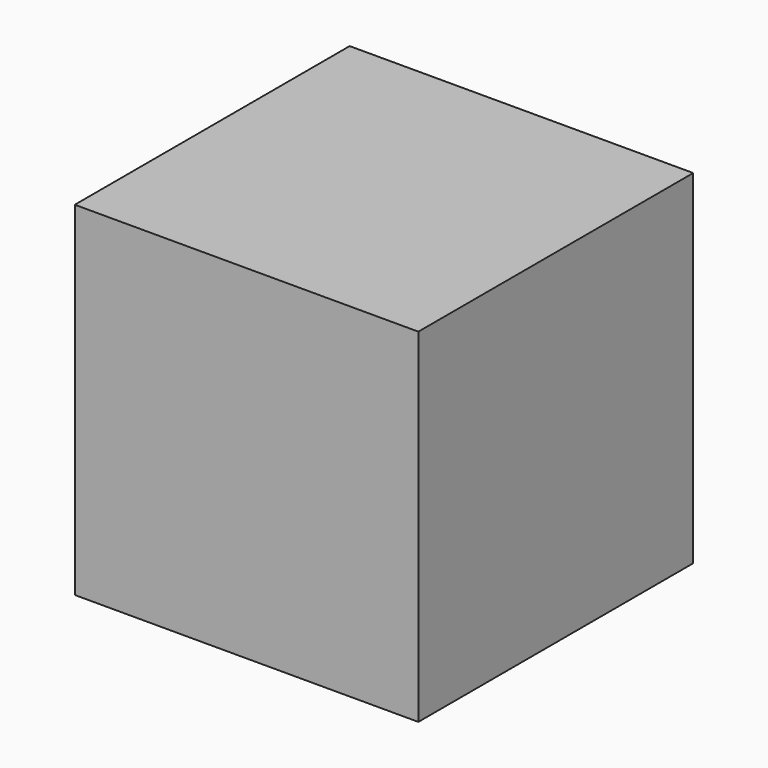
from build123d import *

# Parameters (mm, degrees)
F1_W     = 254
F1_H     = 254
F2_DEPTH = 127


# Not quite as in the source:
# - a variable given as a bare number and used for a length is read in inches; the dataset says mm whatever the document's units were


with BuildPart() as f2:
    # F1 (on Top) → F2 (new body, symmetric)
    with BuildSketch(Plane.XY):
        Rectangle(F1_W, F1_H)
    extrude(amount=F2_DEPTH, both=True)


solid = f2.part
